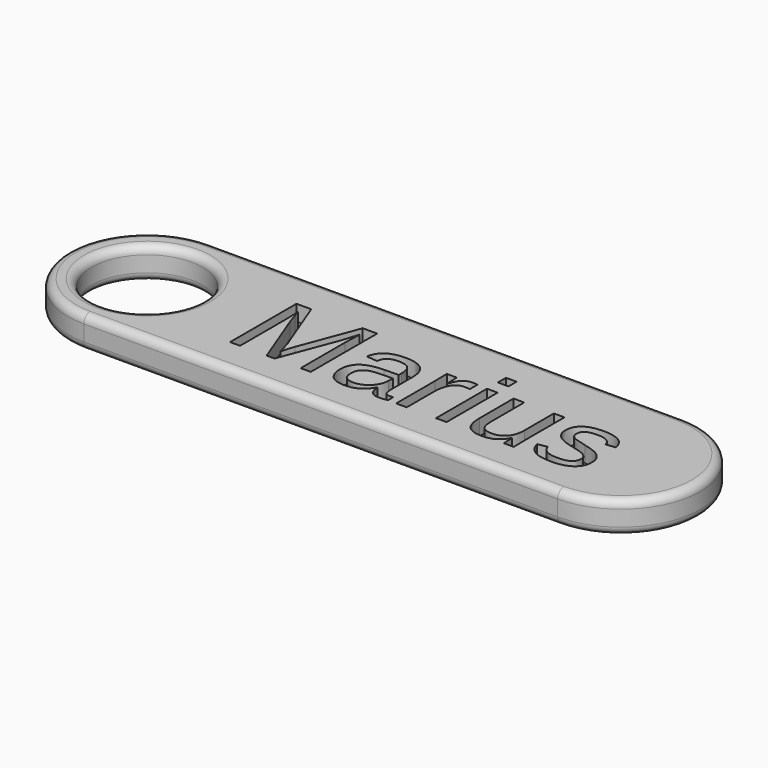
from build123d import *

# Parameters (mm, degrees)
F0_R         = 8.89
F1_DEPTH     = 5.08
F2_TEXT_SIZE = 19.4027777778
F3_DEPTH     = 2.54
F4_R         = 1.27


# Not quite as in the source:
# - Text() gives the source's letters only with a copy of the font that has no kerning and outlines rounded to 1/6400 em; it was checked with that copy


with BuildPart() as f1:
    # F0 (on Top) → F1 (new body)
    with BuildSketch(Plane.XY):
        with BuildLine():
            Line((-38.1, -12.7), (38.1, -12.7))
            ThreePointArc((38.1, -12.7), (50.8, 0), (38.1, 12.7))
            Line((38.1, 12.7), (-38.1, 12.7))
            ThreePointArc((-38.1, 12.7), (-50.8, 0), (-38.1, -12.7))
        make_face()
        with Locations((-38.1, 0)):
            Circle(F0_R, mode=Mode.SUBTRACT)
    extrude(amount=F1_DEPTH)

    # F2 (on face) → F3 (cut)
    with BuildSketch(Plane.XY.offset(5.08)):
        with Locations((-20.7601453993, -6.985)):
            Text('Marius', F2_TEXT_SIZE, font='Arimo', text_align=(TextAlign.LEFT, TextAlign.BOTTOM))
    extrude(amount=-F3_DEPTH, mode=Mode.SUBTRACT)

    # F4
    f4_edges = [f1.edges().sort_by_distance(p)[0] for p in [
        (-50.8, 0, 5.08),
        (0, -12.7, 0),
        (50.8, 0, 0),
        (0, 12.7, 0),
        (-50.8, 0, 0),
        (-46.99, 0, 0),
        (-46.99, 0, 5.08),
    ]]
    fillet(f4_edges, radius=F4_R)


solid = f1.part
